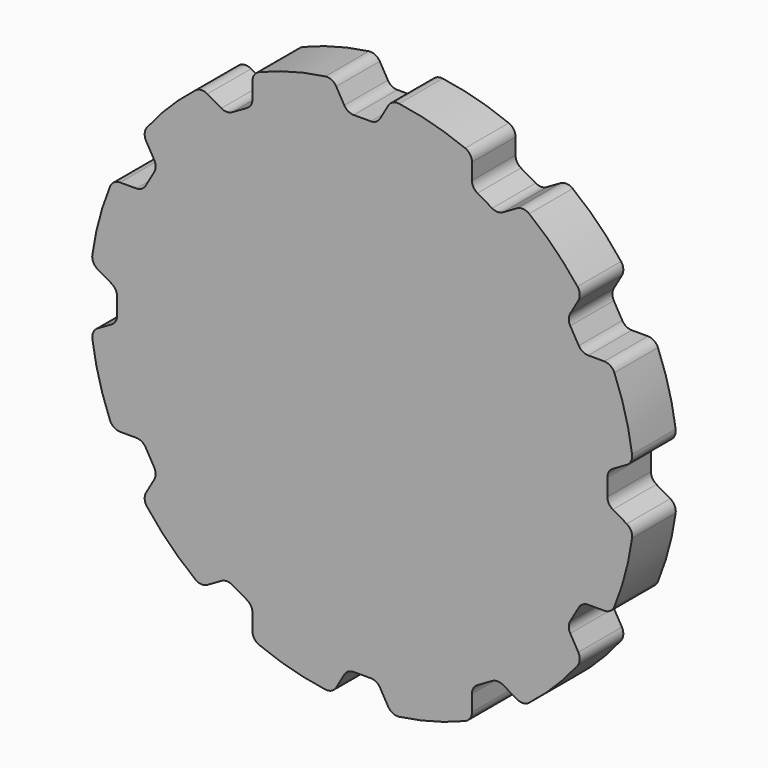
from build123d import *

# Parameters (mm, degrees)
F0_R            = 127
F1_DEPTH        = 12.7
F3_DEPTH        = 12.701
F3_DEPTH_BACK   = 12.701
F3_COPIES_COUNT = 12
F4_T1_DEPTH     = 25.4
F4_T3_DEPTH     = 42.5595323233


# Not quite as in the source:
# - a fillet or chamfer that OpenCascade refuses, or shapes differently, is made with other operations: its cross-section is extruded or revolved along the edge and cut away or added
# - a feature of the source that left no trace in its solid (it failed there, or was rolled back) is left out
# - a pattern or mirror of a feature is missing from the dataset's text; its kind, count and spacing are read off the source's solid


with BuildPart() as f1:
    # F0 (on Front) → F1 (new body, symmetric)
    with BuildSketch(Plane.XZ):
        Circle(F0_R)
    extrude(amount=F1_DEPTH, both=True)

    # F2 (on Front) → F3 (cut, two sides)
    with BuildSketch(Plane.XZ) as f3_sk:
        with BuildLine():
            Line((0, 114.3), (6.8983899217, 114.3))
            Line((6.8983899217, 114.3), (13.7967798433, 126.2483618347))
            ThreePointArc((13.7967798433, 126.2483618347), (0, 127), (-13.7967798433, 126.2483618347))
            Line((-13.7967798433, 126.2483618347), (-6.8983899217, 114.3))
            Line((-6.8983899217, 114.3), (0, 114.3))
        make_face()
    f3 = extrude(amount=-F3_DEPTH, mode=Mode.SUBTRACT) + extrude(f3_sk.sketch, amount=F3_DEPTH_BACK, mode=Mode.SUBTRACT)

    # F3_copies: F3 ×12 about axis
    f3_copies_axis = Axis((0, 0, 0), (0, 1, 0))
    for i in range(1, F3_COPIES_COUNT):
        add(f3.rotate(f3_copies_axis, i * 360 / F3_COPIES_COUNT), mode=Mode.SUBTRACT)

    # F4: fillet of radius 5.08 on 48 edges, made by hand

    # F4_s2 → F4_t1 (join)
    with BuildSketch(Plane.XZ.offset(-12.7)):
        with BuildLine():
            ThreePointArc((8.3648596054, 116.84), (6.5054505542, 114.9805909488), (3.9654505542, 114.3))
            Line((3.9654505542, 114.3), (6.8983899217, 114.3))
            Line((6.8983899217, 114.3), (8.3648596054, 116.84))
        make_face()
        with BuildLine():
            ThreePointArc((-3.9654505542, 114.3), (-6.5054505542, 114.9805909488), (-8.3648596054, 116.84))
            Line((-8.3648596054, 116.84), (-6.8983899217, 114.3))
            Line((-6.8983899217, 114.3), (-3.9654505542, 114.3))
        make_face()
        with BuildLine():
            ThreePointArc((51.1758190826, 105.3688379809), (51.8564100314, 102.8288379809), (53.7158190826, 100.9694289297))
            Line((53.7158190826, 100.9694289297), (51.1758190826, 102.4358986134))
            Line((51.1758190826, 102.4358986134), (51.1758190826, 105.3688379809))
        make_face()
        with BuildLine():
            ThreePointArc((60.5841809174, 97.0039783755), (63.1241809174, 96.3233874267), (65.6641809174, 97.0039783755))
            Line((65.6641809174, 97.0039783755), (63.1241809174, 95.5375086917))
            Line((63.1241809174, 95.5375086917), (60.5841809174, 97.0039783755))
        make_face()
        with BuildLine():
            ThreePointArc((97.0039783755, 65.6641809174), (96.3233874267, 63.1241809174), (97.0039783755, 60.5841809174))
            Line((97.0039783755, 60.5841809174), (95.5375086917, 63.1241809174))
            Line((95.5375086917, 63.1241809174), (97.0039783755, 65.6641809174))
        make_face()
        with BuildLine():
            ThreePointArc((100.9694289297, 53.7158190826), (102.8288379809, 51.8564100314), (105.3688379809, 51.1758190826))
            Line((105.3688379809, 51.1758190826), (102.4358986134, 51.1758190826))
            Line((102.4358986134, 51.1758190826), (100.9694289297, 53.7158190826))
        make_face()
        with BuildLine():
            ThreePointArc((116.84, 8.3648596054), (114.9805909488, 6.5054505542), (114.3, 3.9654505542))
            Line((114.3, 3.9654505542), (114.3, 6.8983899217))
            Line((114.3, 6.8983899217), (116.84, 8.3648596054))
        make_face()
        with BuildLine():
            ThreePointArc((114.3, -3.9654505542), (114.9805909488, -6.5054505542), (116.84, -8.3648596054))
            Line((116.84, -8.3648596054), (114.3, -6.8983899217))
            Line((114.3, -6.8983899217), (114.3, -3.9654505542))
        make_face()
        with BuildLine():
            ThreePointArc((105.3688379809, -51.1758190826), (102.8288379809, -51.8564100314), (100.9694289297, -53.7158190826))
            Line((100.9694289297, -53.7158190826), (102.4358986134, -51.1758190826))
            Line((102.4358986134, -51.1758190826), (105.3688379809, -51.1758190826))
        make_face()
        with BuildLine():
            ThreePointArc((97.0039783755, -60.5841809174), (96.3233874267, -63.1241809174), (97.0039783755, -65.6641809174))
            Line((97.0039783755, -65.6641809174), (95.5375086917, -63.1241809174))
            Line((95.5375086917, -63.1241809174), (97.0039783755, -60.5841809174))
        make_face()
        with BuildLine():
            ThreePointArc((65.6641809174, -97.0039783755), (63.1241809174, -96.3233874267), (60.5841809174, -97.0039783755))
            Line((60.5841809174, -97.0039783755), (63.1241809174, -95.5375086917))
            Line((63.1241809174, -95.5375086917), (65.6641809174, -97.0039783755))
        make_face()
        with BuildLine():
            ThreePointArc((53.7158190826, -100.9694289297), (51.8564100314, -102.8288379809), (51.1758190826, -105.3688379809))
            Line((51.1758190826, -105.3688379809), (51.1758190826, -102.4358986134))
            Line((51.1758190826, -102.4358986134), (53.7158190826, -100.9694289297))
        make_face()
        with BuildLine():
            ThreePointArc((8.3648596054, -116.84), (6.5054505542, -114.9805909488), (3.9654505542, -114.3))
            Line((3.9654505542, -114.3), (6.8983899217, -114.3))
            Line((6.8983899217, -114.3), (8.3648596054, -116.84))
        make_face()
        with BuildLine():
            ThreePointArc((-3.9654505542, -114.3), (-6.5054505542, -114.9805909488), (-8.3648596054, -116.84))
            Line((-8.3648596054, -116.84), (-6.8983899217, -114.3))
            Line((-6.8983899217, -114.3), (-3.9654505542, -114.3))
        make_face()
        with BuildLine():
            ThreePointArc((-51.1758190826, -105.3688379809), (-51.8564100314, -102.8288379809), (-53.7158190826, -100.9694289297))
            Line((-53.7158190826, -100.9694289297), (-51.1758190826, -102.4358986134))
            Line((-51.1758190826, -102.4358986134), (-51.1758190826, -105.3688379809))
        make_face()
        with BuildLine():
            ThreePointArc((-60.5841809174, -97.0039783755), (-63.1241809174, -96.3233874267), (-65.6641809174, -97.0039783755))
            Line((-65.6641809174, -97.0039783755), (-63.1241809174, -95.5375086917))
            Line((-63.1241809174, -95.5375086917), (-60.5841809174, -97.0039783755))
        make_face()
        with BuildLine():
            ThreePointArc((-97.0039783755, -65.6641809174), (-96.3233874267, -63.1241809174), (-97.0039783755, -60.5841809174))
            Line((-97.0039783755, -60.5841809174), (-95.5375086917, -63.1241809174))
            Line((-95.5375086917, -63.1241809174), (-97.0039783755, -65.6641809174))
        make_face()
        with BuildLine():
            ThreePointArc((-100.9694289297, -53.7158190826), (-102.8288379809, -51.8564100314), (-105.3688379809, -51.1758190826))
            Line((-105.3688379809, -51.1758190826), (-102.4358986134, -51.1758190826))
            Line((-102.4358986134, -51.1758190826), (-100.9694289297, -53.7158190826))
        make_face()
        with BuildLine():
            ThreePointArc((-116.84, -8.3648596054), (-114.9805909488, -6.5054505542), (-114.3, -3.9654505542))
            Line((-114.3, -3.9654505542), (-114.3, -6.8983899217))
            Line((-114.3, -6.8983899217), (-116.84, -8.3648596054))
        make_face()
        with BuildLine():
            ThreePointArc((-114.3, 3.9654505542), (-114.9805909488, 6.5054505542), (-116.84, 8.3648596054))
            Line((-116.84, 8.3648596054), (-114.3, 6.8983899217))
            Line((-114.3, 6.8983899217), (-114.3, 3.9654505542))
        make_face()
        with BuildLine():
            ThreePointArc((-105.3688379809, 51.1758190826), (-102.8288379809, 51.8564100314), (-100.9694289297, 53.7158190826))
            Line((-100.9694289297, 53.7158190826), (-102.4358986134, 51.1758190826))
            Line((-102.4358986134, 51.1758190826), (-105.3688379809, 51.1758190826))
        make_face()
        with BuildLine():
            ThreePointArc((-97.0039783755, 60.5841809174), (-96.3233874267, 63.1241809174), (-97.0039783755, 65.6641809174))
            Line((-97.0039783755, 65.6641809174), (-95.5375086917, 63.1241809174))
            Line((-95.5375086917, 63.1241809174), (-97.0039783755, 60.5841809174))
        make_face()
        with BuildLine():
            ThreePointArc((-65.6641809174, 97.0039783755), (-63.1241809174, 96.3233874267), (-60.5841809174, 97.0039783755))
            Line((-60.5841809174, 97.0039783755), (-63.1241809174, 95.5375086917))
            Line((-63.1241809174, 95.5375086917), (-65.6641809174, 97.0039783755))
        make_face()
        with BuildLine():
            ThreePointArc((-53.7158190826, 100.9694289297), (-51.8564100314, 102.8288379809), (-51.1758190826, 105.3688379809))
            Line((-51.1758190826, 105.3688379809), (-51.1758190826, 102.4358986134))
            Line((-51.1758190826, 102.4358986134), (-53.7158190826, 100.9694289297))
        make_face()
    extrude(amount=F4_T1_DEPTH)

    # F4_s4 → F4_t3 (cut)
    with BuildSketch(Plane.XZ.offset(-21.2797661616)):
        with BuildLine():
            ThreePointArc((17.2030259978, 125.8294714942), (14.2794184599, 125.3579809313), (12.1154959066, 123.3362926345))
            Line((12.1154959066, 123.3362926345), (13.7967798433, 126.2483618347))
            ThreePointArc((13.7967798433, 126.2483618347), (15.5013179384, 126.0504230147), (17.2030259978, 125.8294714942))
        make_face()
        with BuildLine():
            ThreePointArc((-12.1154959066, 123.3362926345), (-14.2794184599, 125.3579809313), (-17.2030259978, 125.8294714942))
            ThreePointArc((-17.2030259978, 125.8294714942), (-15.5013179384, 126.0504230147), (-13.7967798433, 126.2483618347))
            Line((-13.7967798433, 126.2483618347), (-12.1154959066, 123.3362926345))
        make_face()
        with BuildLine():
            ThreePointArc((48.0164782111, 117.5730318577), (50.3126513281, 115.7029052836), (51.1758190826, 112.8701105834))
            Line((51.1758190826, 112.8701105834), (51.1758190826, 116.2326784567))
            ThreePointArc((51.1758190826, 116.2326784567), (49.6006763806, 116.9135274576), (48.0164782111, 117.5730318577))
        make_face()
        with BuildLine():
            ThreePointArc((72.1604735518, 100.7546146767), (75.0453296032, 101.4234868237), (77.8129932832, 100.3700058599))
            ThreePointArc((77.8129932832, 100.3700058599), (76.4497466341, 101.4122095193), (75.0725427521, 102.4358986134))
            Line((75.0725427521, 102.4358986134), (72.1604735518, 100.7546146767))
        make_face()
        with BuildLine():
            ThreePointArc((100.3700058599, 77.8129932832), (101.4234868237, 75.0453296032), (100.7546146767, 72.1604735518))
            Line((100.7546146767, 72.1604735518), (102.4358986134, 75.0725427521))
            ThreePointArc((102.4358986134, 75.0725427521), (101.4122095193, 76.4497466341), (100.3700058599, 77.8129932832))
        make_face()
        with BuildLine():
            ThreePointArc((112.8701105834, 51.1758190826), (115.7029052836, 50.3126513281), (117.5730318577, 48.0164782111))
            ThreePointArc((117.5730318577, 48.0164782111), (116.9135274576, 49.6006763806), (116.2326784567, 51.1758190826))
            Line((116.2326784567, 51.1758190826), (112.8701105834, 51.1758190826))
        make_face()
        with BuildLine():
            ThreePointArc((125.8294714942, 17.2030259978), (125.3579809313, 14.2794184599), (123.3362926345, 12.1154959067))
            Line((123.3362926345, 12.1154959067), (126.2483618347, 13.7967798433))
            ThreePointArc((126.2483618347, 13.7967798433), (126.0504230147, 15.5013179384), (125.8294714942, 17.2030259978))
        make_face()
        with BuildLine():
            ThreePointArc((123.3362926345, -12.1154959066), (125.3579809313, -14.2794184599), (125.8294714942, -17.2030259978))
            ThreePointArc((125.8294714942, -17.2030259978), (126.0504230147, -15.5013179384), (126.2483618347, -13.7967798433))
            Line((126.2483618347, -13.7967798433), (123.3362926345, -12.1154959066))
        make_face()
        with BuildLine():
            ThreePointArc((117.5730318577, -48.0164782111), (115.7029052836, -50.3126513281), (112.8701105834, -51.1758190826))
            Line((112.8701105834, -51.1758190826), (116.2326784567, -51.1758190826))
            ThreePointArc((116.2326784567, -51.1758190826), (116.9135274576, -49.6006763806), (117.5730318577, -48.0164782111))
        make_face()
        with BuildLine():
            ThreePointArc((100.7546146767, -72.1604735518), (101.4234868237, -75.0453296032), (100.3700058599, -77.8129932832))
            ThreePointArc((100.3700058599, -77.8129932832), (101.4122095193, -76.4497466341), (102.4358986134, -75.0725427521))
            Line((102.4358986134, -75.0725427521), (100.7546146767, -72.1604735518))
        make_face()
        with BuildLine():
            ThreePointArc((77.8129932832, -100.3700058599), (75.0453296032, -101.4234868237), (72.1604735518, -100.7546146767))
            Line((72.1604735518, -100.7546146767), (75.0725427521, -102.4358986134))
            ThreePointArc((75.0725427521, -102.4358986134), (76.4497466341, -101.4122095193), (77.8129932832, -100.3700058599))
        make_face()
        with BuildLine():
            ThreePointArc((51.1758190826, -112.8701105834), (50.3126513281, -115.7029052836), (48.0164782111, -117.5730318577))
            ThreePointArc((48.0164782111, -117.5730318577), (49.6006763806, -116.9135274576), (51.1758190826, -116.2326784567))
            Line((51.1758190826, -116.2326784567), (51.1758190826, -112.8701105834))
        make_face()
        with BuildLine():
            ThreePointArc((17.2030259978, -125.8294714942), (14.2794184599, -125.3579809313), (12.1154959067, -123.3362926345))
            Line((12.1154959067, -123.3362926345), (13.7967798433, -126.2483618347))
            ThreePointArc((13.7967798433, -126.2483618347), (15.5013179384, -126.0504230147), (17.2030259978, -125.8294714942))
        make_face()
        with BuildLine():
            ThreePointArc((-12.1154959066, -123.3362926345), (-14.2794184599, -125.3579809313), (-17.2030259978, -125.8294714942))
            ThreePointArc((-17.2030259978, -125.8294714942), (-15.5013179384, -126.0504230147), (-13.7967798433, -126.2483618347))
            Line((-13.7967798433, -126.2483618347), (-12.1154959066, -123.3362926345))
        make_face()
        with BuildLine():
            ThreePointArc((-48.0164782111, -117.5730318577), (-50.3126513281, -115.7029052836), (-51.1758190826, -112.8701105834))
            Line((-51.1758190826, -112.8701105834), (-51.1758190826, -116.2326784567))
            ThreePointArc((-51.1758190826, -116.2326784567), (-49.6006763806, -116.9135274576), (-48.0164782111, -117.5730318577))
        make_face()
        with BuildLine():
            ThreePointArc((-72.1604735518, -100.7546146767), (-75.0453296032, -101.4234868237), (-77.8129932832, -100.3700058599))
            ThreePointArc((-77.8129932832, -100.3700058599), (-76.4497466341, -101.4122095193), (-75.0725427521, -102.4358986134))
            Line((-75.0725427521, -102.4358986134), (-72.1604735518, -100.7546146767))
        make_face()
        with BuildLine():
            ThreePointArc((-100.3700058599, -77.8129932832), (-101.4234868237, -75.0453296032), (-100.7546146767, -72.1604735518))
            Line((-100.7546146767, -72.1604735518), (-102.4358986134, -75.0725427521))
            ThreePointArc((-102.4358986134, -75.0725427521), (-101.4122095193, -76.4497466341), (-100.3700058599, -77.8129932832))
        make_face()
        with BuildLine():
            ThreePointArc((-112.8701105834, -51.1758190826), (-115.7029052836, -50.3126513281), (-117.5730318577, -48.0164782111))
            ThreePointArc((-117.5730318577, -48.0164782111), (-116.9135274576, -49.6006763806), (-116.2326784567, -51.1758190826))
            Line((-116.2326784567, -51.1758190826), (-112.8701105834, -51.1758190826))
        make_face()
        with BuildLine():
            ThreePointArc((-125.8294714942, -17.2030259978), (-125.3579809313, -14.2794184599), (-123.3362926345, -12.1154959066))
            Line((-123.3362926345, -12.1154959066), (-126.2483618347, -13.7967798433))
            ThreePointArc((-126.2483618347, -13.7967798433), (-126.0504230147, -15.5013179384), (-125.8294714942, -17.2030259978))
        make_face()
        with BuildLine():
            ThreePointArc((-123.3362926345, 12.1154959066), (-125.3579809313, 14.2794184599), (-125.8294714942, 17.2030259978))
            ThreePointArc((-125.8294714942, 17.2030259978), (-126.0504230147, 15.5013179384), (-126.2483618347, 13.7967798433))
            Line((-126.2483618347, 13.7967798433), (-123.3362926345, 12.1154959066))
        make_face()
        with BuildLine():
            ThreePointArc((-117.5730318577, 48.0164782111), (-115.7029052836, 50.3126513281), (-112.8701105834, 51.1758190826))
            Line((-112.8701105834, 51.1758190826), (-116.2326784567, 51.1758190826))
            ThreePointArc((-116.2326784567, 51.1758190826), (-116.9135274576, 49.6006763806), (-117.5730318577, 48.0164782111))
        make_face()
        with BuildLine():
            ThreePointArc((-100.7546146767, 72.1604735518), (-101.4234868237, 75.0453296032), (-100.3700058599, 77.8129932832))
            ThreePointArc((-100.3700058599, 77.8129932832), (-101.4122095193, 76.4497466341), (-102.4358986134, 75.0725427521))
            Line((-102.4358986134, 75.0725427521), (-100.7546146767, 72.1604735518))
        make_face()
        with BuildLine():
            ThreePointArc((-77.8129932832, 100.3700058599), (-75.0453296032, 101.4234868237), (-72.1604735518, 100.7546146767))
            Line((-72.1604735518, 100.7546146767), (-75.0725427521, 102.4358986134))
            ThreePointArc((-75.0725427521, 102.4358986134), (-76.4497466341, 101.4122095193), (-77.8129932832, 100.3700058599))
        make_face()
        with BuildLine():
            ThreePointArc((-51.1758190826, 112.8701105834), (-50.3126513281, 115.7029052836), (-48.0164782111, 117.5730318577))
            ThreePointArc((-48.0164782111, 117.5730318577), (-49.6006763806, 116.9135274576), (-51.1758190826, 116.2326784567))
            Line((-51.1758190826, 116.2326784567), (-51.1758190826, 112.8701105834))
        make_face()
    extrude(amount=F4_T3_DEPTH, mode=Mode.SUBTRACT)


solid = f1.part
